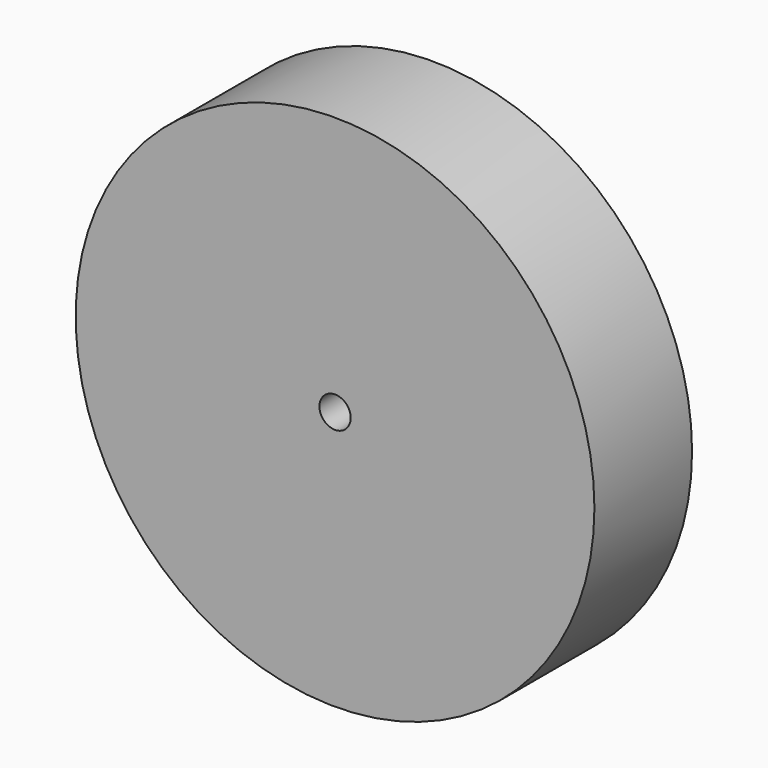
from build123d import *

# Parameters (mm, degrees)
F0_R     = 26.9875
F0_R_2   = 1.6256
F1_DEPTH = 12.7


# Not quite as in the source:
# - a feature names something its author has since deleted; it is built from what else it names


with BuildPart() as f1:
    # F0 (on Front) → F1 (new body)
    with BuildSketch(Plane.XZ):
        Circle(F0_R)
        Circle(F0_R_2, mode=Mode.SUBTRACT)
    extrude(amount=F1_DEPTH)


solid = f1.part
